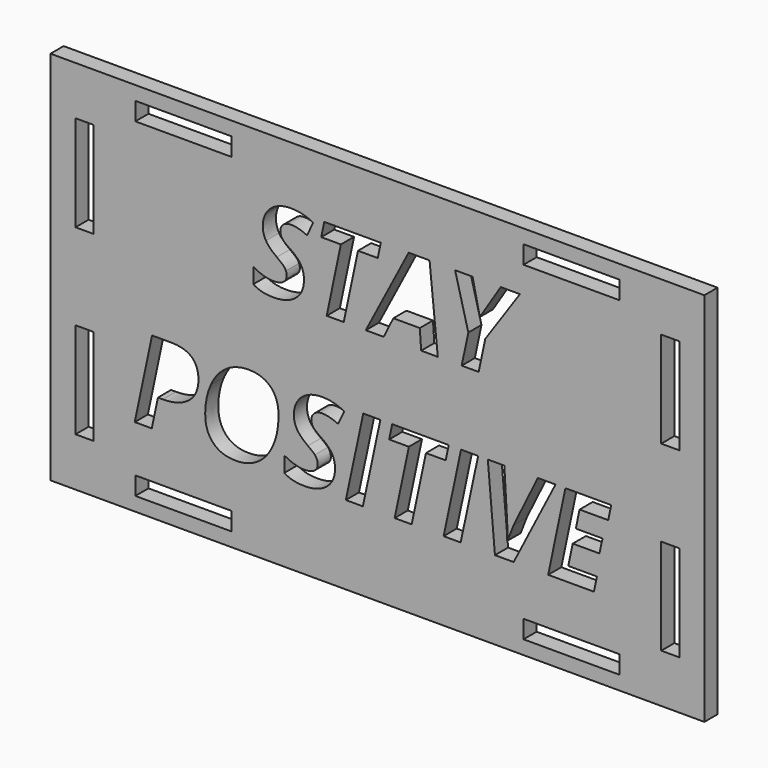
from build123d import *

# Parameters (mm, degrees)
F0_W     = 119.38
F0_H     = 68.58
F0_W_2   = 17.526
F0_H_2   = 3.302
F0_W_3   = 3.302
F0_H_3   = 17.526
F1_DEPTH = 3


with BuildPart() as f1:
    # F0 (on Front) → F1 (new body)
    with BuildSketch(Plane.XZ):
        Rectangle(F0_W, F0_H)
        with Locations((-35.433, -30.099)):
            Rectangle(F0_W_2, F0_H_2, mode=Mode.SUBTRACT)
        with Locations((-53.467, -16.637)):
            Rectangle(F0_W_3, F0_H_3, mode=Mode.SUBTRACT)
        with BuildLine():
            add(Edge.make_bspline(
                [(-33.9483112605, -6.0585155259), (-32.6803680163, -7.148128688), (-32.6803680163, -9.3240829005)],
                knots=[0, 0, 0, 1, 1, 1], degree=2))
            add(Edge.make_bspline(
                [(-32.6803680163, -9.3240829005), (-32.6803680163, -11.7912550452), (-34.4145871632, -13.1966269765)],
                knots=[0, 0, 0, 1, 1, 1], degree=2))
            add(Edge.make_bspline(
                [(-34.4145871632, -13.1966269765), (-36.14880631, -14.6019989077), (-39.1951422075, -14.6019989077)],
                knots=[0, 0, 0, 1, 1, 1], degree=2))
            Line((-39.1951422075, -14.6019989077), (-40.0753402273, -14.6019989077))
            Line((-40.0753402273, -14.6019989077), (-41.1878581706, -19.9191802541))
            Line((-41.1878581706, -19.9191802541), (-44.3061805232, -19.9191802541))
            Line((-44.3061805232, -19.9191802541), (-41.1485928314, -4.9689023639))
            Line((-41.1485928314, -4.9689023639), (-37.6899708725, -4.9689023639))
            add(Edge.make_bspline(
                [(-37.6899708725, -4.9689023639), (-35.2162545046, -4.9689023639), (-33.9483112605, -6.0585155259)],
                knots=[0, 0, 0, 1, 1, 1], degree=2))
        make_face(mode=Mode.SUBTRACT)
        with BuildLine():
            add(Edge.make_bspline(
                [(-19.4888501099, -6.2057605478), (-18.0573012859, -7.6782107668), (-18.0573012859, -10.328621161)],
                knots=[0, 0, 0, 1, 1, 1], degree=2))
            add(Edge.make_bspline(
                [(-18.0573012859, -10.328621161), (-18.0573012859, -13.2211678135), (-19.0700198254, -15.5067377645)],
                knots=[0, 0, 0, 1, 1, 1], degree=2))
            add(Edge.make_bspline(
                [(-19.0700198254, -15.5067377645), (-20.0827383649, -17.7923077156), (-21.8414983487, -18.9588155002)],
                knots=[0, 0, 0, 1, 1, 1], degree=2))
            add(Edge.make_bspline(
                [(-21.8414983487, -18.9588155002), (-23.6002583325, -20.1253232848), (-25.890736451, -20.1253232848)],
                knots=[0, 0, 0, 1, 1, 1], degree=2))
            add(Edge.make_bspline(
                [(-25.890736451, -20.1253232848), (-28.5084257292, -20.1253232848), (-29.9759677808, -18.6168798382)],
                knots=[0, 0, 0, 1, 1, 1], degree=2))
            add(Edge.make_bspline(
                [(-29.9759677808, -18.6168798382), (-31.4435098324, -17.1084363916), (-31.4435098324, -14.428576993)],
                knots=[0, 0, 0, 1, 1, 1], degree=2))
            add(Edge.make_bspline(
                [(-31.4435098324, -14.428576993), (-31.4435098324, -11.7192685901), (-30.4307912929, -9.4435149738)],
                knots=[0, 0, 0, 1, 1, 1], degree=2))
            add(Edge.make_bspline(
                [(-30.4307912929, -9.4435149738), (-29.4180727534, -7.1677613576), (-27.6380440442, -5.9505358432)],
                knots=[0, 0, 0, 1, 1, 1], degree=2))
            add(Edge.make_bspline(
                [(-27.6380440442, -5.9505358432), (-25.858015335, -4.7333103288), (-23.5282718774, -4.7333103288)],
                knots=[0, 0, 0, 1, 1, 1], degree=2))
            add(Edge.make_bspline(
                [(-23.5282718774, -4.7333103288), (-20.9203989339, -4.7333103288), (-19.4888501099, -6.2057605478)],
                knots=[0, 0, 0, 1, 1, 1], degree=2))
        make_face(mode=Mode.SUBTRACT)
        with BuildLine():
            add(Edge.make_bspline(
                [(-8.3538543427, -13.1966269765), (-7.7403334181, -14.1831686232), (-7.7403334181, -15.5018295971)],
                knots=[0, 0, 0, 1, 1, 1], degree=2))
            add(Edge.make_bspline(
                [(-7.7403334181, -15.5018295971), (-7.7403334181, -17.6385184705), (-9.2536850321, -18.8819208776)],
                knots=[0, 0, 0, 1, 1, 1], degree=2))
            add(Edge.make_bspline(
                [(-9.2536850321, -18.8819208776), (-10.767036646, -20.1253232848), (-13.3520048083, -20.1253232848)],
                knots=[0, 0, 0, 1, 1, 1], degree=2))
            add(Edge.make_bspline(
                [(-13.3520048083, -20.1253232848), (-15.6130339223, -20.1253232848), (-16.9938650166, -19.2025878142)],
                knots=[0, 0, 0, 1, 1, 1], degree=2))
            Line((-16.9938650166, -19.2025878142), (-16.9938650166, -16.4016602865))
            add(Edge.make_bspline(
                [(-16.9938650166, -16.4016602865), (-15.0207817231, -17.504361895), (-13.3323721387, -17.504361895)],
                knots=[0, 0, 0, 1, 1, 1], degree=2))
            add(Edge.make_bspline(
                [(-13.3323721387, -17.504361895), (-12.1871330795, -17.504361895), (-11.5425270947, -17.0708071083)],
                knots=[0, 0, 0, 1, 1, 1], degree=2))
            add(Edge.make_bspline(
                [(-11.5425270947, -17.0708071083), (-10.8979211099, -16.6372523215), (-10.8979211099, -15.8813945425)],
                knots=[0, 0, 0, 1, 1, 1], degree=2))
            add(Edge.make_bspline(
                [(-10.8979211099, -15.8813945425), (-10.8979211099, -15.4396594768), (-11.0369858528, -15.1075401496)],
                knots=[0, 0, 0, 1, 1, 1], degree=2))
            add(Edge.make_bspline(
                [(-11.0369858528, -15.1075401496), (-11.1760505957, -14.7754208224), (-11.4312753004, -14.4891110576)],
                knots=[0, 0, 0, 1, 1, 1], degree=2))
            add(Edge.make_bspline(
                [(-11.4312753004, -14.4891110576), (-11.686500005, -14.2028012928), (-12.6975824887, -13.4469435137)],
                knots=[0, 0, 0, 1, 1, 1], degree=2))
            add(Edge.make_bspline(
                [(-12.6975824887, -13.4469435137), (-14.111134699, -12.4325889184), (-14.6837542286, -11.4411391043)],
                knots=[0, 0, 0, 1, 1, 1], degree=2))
            add(Edge.make_bspline(
                [(-14.6837542286, -11.4411391043), (-15.2563737582, -10.4496892902), (-15.2563737582, -9.3044502309)],
                knots=[0, 0, 0, 1, 1, 1], degree=2))
            add(Edge.make_bspline(
                [(-15.2563737582, -9.3044502309), (-15.2563737582, -7.985789257), (-14.6215841082, -6.9485298805)],
                knots=[0, 0, 0, 1, 1, 1], degree=2))
            add(Edge.make_bspline(
                [(-14.6215841082, -6.9485298805), (-13.9867944582, -5.911270504), (-12.8153785062, -5.333742807)],
                knots=[0, 0, 0, 1, 1, 1], degree=2))
            add(Edge.make_bspline(
                [(-12.8153785062, -5.333742807), (-11.6439625542, -4.75621511), (-10.1224306613, -4.75621511)],
                knots=[0, 0, 0, 1, 1, 1], degree=2))
            add(Edge.make_bspline(
                [(-10.1224306613, -4.75621511), (-7.903938998, -4.75621511), (-6.0617401684, -5.7672975937)],
                knots=[0, 0, 0, 1, 1, 1], degree=2))
            Line((-6.0617401684, -5.7672975937), (-7.1775302233, -8.1493948369))
            add(Edge.make_bspline(
                [(-7.1775302233, -8.1493948369), (-8.7710485714, -7.3935370578), (-10.1224306613, -7.3935370578)],
                knots=[0, 0, 0, 1, 1, 1], degree=2))
            add(Edge.make_bspline(
                [(-10.1224306613, -7.3935370578), (-10.9699075651, -7.3935370578), (-11.5114420345, -7.8532687373)],
                knots=[0, 0, 0, 1, 1, 1], degree=2))
            add(Edge.make_bspline(
                [(-11.5114420345, -7.8532687373), (-12.052976504, -8.3130004168), (-12.052976504, -9.0688581959)],
                knots=[0, 0, 0, 1, 1, 1], degree=2))
            add(Edge.make_bspline(
                [(-12.052976504, -9.0688581959), (-12.052976504, -9.6938315111), (-11.7159490094, -10.1584713579)],
                knots=[0, 0, 0, 1, 1, 1], degree=2))
            add(Edge.make_bspline(
                [(-11.7159490094, -10.1584713579), (-11.3789215148, -10.6231112048), (-10.2042334512, -11.3920574303)],
                knots=[0, 0, 0, 1, 1, 1], degree=2))
            add(Edge.make_bspline(
                [(-10.2042334512, -11.3920574303), (-8.9673752672, -12.2100853298), (-8.3538543427, -13.1966269765)],
                knots=[0, 0, 0, 1, 1, 1], degree=2))
        make_face(mode=Mode.SUBTRACT)
        Polygon((-2.6554719951, -19.9191802541), (-5.7737943478, -19.9191802541), (-2.58348554, -4.9689023639), (0.5348368127, -4.9689023639), align=None, mode=Mode.SUBTRACT)
        with Locations((35.433, -30.099)):
            Rectangle(F0_W_2, F0_H_2, mode=Mode.SUBTRACT)
        Polygon((8.8558166058, -7.6062243117), (6.2577599972, -19.9191802541), (3.1394376445, -19.9191802541), (5.7374942532, -7.6062243117), (2.1381714956, -7.6062243117), (2.7009746904, -4.9689023639), (13.027758893, -4.9689023639), (12.4649556982, -7.6062243117), align=None, mode=Mode.SUBTRACT)
        Polygon((15.1971688823, -19.9191802541), (12.0788465297, -19.9191802541), (15.2691553375, -4.9689023639), (18.3874776902, -4.9689023639), align=None, mode=Mode.SUBTRACT)
        with BuildLine():
            Line((23.6719379206, -16.8630280218), (23.7439243757, -16.8630280218))
            add(Edge.make_bspline(
                [(23.7439243757, -16.8630280218), (24.5423196056, -14.6019989077), (24.8695307654, -13.9672092578)],
                knots=[0, 0, 0, 1, 1, 1], degree=2))
            Line((24.8695307654, -13.9672092578), (29.2868814224, -4.9689023639))
            Line((29.2868814224, -4.9689023639), (32.5164555694, -4.9689023639))
            Line((32.5164555694, -4.9689023639), (24.8695307654, -19.9191802541))
            Line((24.8695307654, -19.9191802541), (21.4534462573, -19.9191802541))
            Line((21.4534462573, -19.9191802541), (20.154417953, -4.9689023639))
            Line((20.154417953, -4.9689023639), (23.1713048461, -4.9689023639))
            Line((23.1713048461, -4.9689023639), (23.6915705902, -13.9672092578))
            add(Edge.make_bspline(
                [(23.6915705902, -13.9672092578), (23.7341080409, -14.428576993), (23.7341080409, -15.3284076824)],
                knots=[0, 0, 0, 1, 1, 1], degree=2))
            add(Edge.make_bspline(
                [(23.7341080409, -15.3284076824), (23.7144753713, -16.3820276169), (23.6719379206, -16.8630280218)],
                knots=[0, 0, 0, 1, 1, 1], degree=2))
        make_face(mode=Mode.SUBTRACT)
        Polygon((40.0750333602, -17.3014909759), (39.5220465002, -19.9191802541), (31.1683455911, -19.9191802541), (34.3259332829, -4.9689023639), (42.6927226385, -4.9689023639), (42.1397357784, -7.5669589725), (36.904357222, -7.5669589725), (36.2172137865, -10.8488869051), (41.0959321787, -10.8488869051), (40.5331289839, -13.4469435137), (35.6576827032, -13.4469435137), (34.8396548038, -17.3014909759), align=None, mode=Mode.SUBTRACT)
        with Locations((53.467, -16.637)):
            Rectangle(F0_W_3, F0_H_3, mode=Mode.SUBTRACT)
        with Locations((-53.467, 16.637)):
            Rectangle(F0_W_3, F0_H_3, mode=Mode.SUBTRACT)
        with BuildLine():
            add(Edge.make_bspline(
                [(-14.0244237416, 15.2838323706), (-13.410902817, 14.2972907238), (-13.410902817, 12.9786297499)],
                knots=[0, 0, 0, 1, 1, 1], degree=2))
            add(Edge.make_bspline(
                [(-13.410902817, 12.9786297499), (-13.410902817, 10.8419408766), (-14.924254431, 9.5985384694)],
                knots=[0, 0, 0, 1, 1, 1], degree=2))
            add(Edge.make_bspline(
                [(-14.924254431, 9.5985384694), (-16.437606045, 8.3551360623), (-19.0225742072, 8.3551360623)],
                knots=[0, 0, 0, 1, 1, 1], degree=2))
            add(Edge.make_bspline(
                [(-19.0225742072, 8.3551360623), (-21.2836033213, 8.3551360623), (-22.6644344155, 9.2778715328)],
                knots=[0, 0, 0, 1, 1, 1], degree=2))
            Line((-22.6644344155, 9.2778715328), (-22.6644344155, 12.0787990605))
            add(Edge.make_bspline(
                [(-22.6644344155, 12.0787990605), (-20.6913511221, 10.9760974521), (-19.0029415376, 10.9760974521)],
                knots=[0, 0, 0, 1, 1, 1], degree=2))
            add(Edge.make_bspline(
                [(-19.0029415376, 10.9760974521), (-17.8577024784, 10.9760974521), (-17.2130964936, 11.4096522388)],
                knots=[0, 0, 0, 1, 1, 1], degree=2))
            add(Edge.make_bspline(
                [(-17.2130964936, 11.4096522388), (-16.5684905089, 11.8432070255), (-16.5684905089, 12.5990648046)],
                knots=[0, 0, 0, 1, 1, 1], degree=2))
            add(Edge.make_bspline(
                [(-16.5684905089, 12.5990648046), (-16.5684905089, 13.0407998703), (-16.7075552518, 13.3729191975)],
                knots=[0, 0, 0, 1, 1, 1], degree=2))
            add(Edge.make_bspline(
                [(-16.7075552518, 13.3729191975), (-16.8466199947, 13.7050385246), (-17.1018446993, 13.9913482894)],
                knots=[0, 0, 0, 1, 1, 1], degree=2))
            add(Edge.make_bspline(
                [(-17.1018446993, 13.9913482894), (-17.3570694039, 14.2776580542), (-18.3681518877, 15.0335158333)],
                knots=[0, 0, 0, 1, 1, 1], degree=2))
            add(Edge.make_bspline(
                [(-18.3681518877, 15.0335158333), (-19.7817040979, 16.0478704286), (-20.3543236275, 17.0393202428)],
                knots=[0, 0, 0, 1, 1, 1], degree=2))
            add(Edge.make_bspline(
                [(-20.3543236275, 17.0393202428), (-20.9269431571, 18.0307700569), (-20.9269431571, 19.1760091161)],
                knots=[0, 0, 0, 1, 1, 1], degree=2))
            add(Edge.make_bspline(
                [(-20.9269431571, 19.1760091161), (-20.9269431571, 20.49467009), (-20.2921535072, 21.5319294665)],
                knots=[0, 0, 0, 1, 1, 1], degree=2))
            add(Edge.make_bspline(
                [(-20.2921535072, 21.5319294665), (-19.6573638572, 22.569188843), (-18.4859479052, 23.14671654)],
                knots=[0, 0, 0, 1, 1, 1], degree=2))
            add(Edge.make_bspline(
                [(-18.4859479052, 23.14671654), (-17.3145319532, 23.724244237), (-15.7930000602, 23.724244237)],
                knots=[0, 0, 0, 1, 1, 1], degree=2))
            add(Edge.make_bspline(
                [(-15.7930000602, 23.724244237), (-13.5745083969, 23.724244237), (-11.7323095674, 22.7131617533)],
                knots=[0, 0, 0, 1, 1, 1], degree=2))
            Line((-11.7323095674, 22.7131617533), (-12.8480996222, 20.3310645101))
            add(Edge.make_bspline(
                [(-12.8480996222, 20.3310645101), (-14.4416179703, 21.0869222892), (-15.7930000602, 21.0869222892)],
                knots=[0, 0, 0, 1, 1, 1], degree=2))
            add(Edge.make_bspline(
                [(-15.7930000602, 21.0869222892), (-16.640476964, 21.0869222892), (-17.1820114335, 20.6271906097)],
                knots=[0, 0, 0, 1, 1, 1], degree=2))
            add(Edge.make_bspline(
                [(-17.1820114335, 20.6271906097), (-17.7235459029, 20.1674589302), (-17.7235459029, 19.4116011512)],
                knots=[0, 0, 0, 1, 1, 1], degree=2))
            add(Edge.make_bspline(
                [(-17.7235459029, 19.4116011512), (-17.7235459029, 18.786627836), (-17.3865184083, 18.3219879891)],
                knots=[0, 0, 0, 1, 1, 1], degree=2))
            add(Edge.make_bspline(
                [(-17.3865184083, 18.3219879891), (-17.0494909138, 17.8573481422), (-15.8748028502, 17.0884019167)],
                knots=[0, 0, 0, 1, 1, 1], degree=2))
            add(Edge.make_bspline(
                [(-15.8748028502, 17.0884019167), (-14.6379446662, 16.2703740173), (-14.0244237416, 15.2838323706)],
                knots=[0, 0, 0, 1, 1, 1], degree=2))
        make_face(mode=Mode.SUBTRACT)
        Polygon((-3.5520305729, 20.8742350354), (-6.1500871816, 8.5612790929), (-9.2684095342, 8.5612790929), (-6.6703529256, 20.8742350354), (-10.2696756832, 20.8742350354), (-9.7068724883, 23.5115569832), (0.6199117142, 23.5115569832), (0.0571085194, 20.8742350354), align=None, mode=Mode.SUBTRACT)
        with Locations((-35.433, 30.099)):
            Rectangle(F0_W_2, F0_H_2, mode=Mode.SUBTRACT)
        Polygon((7.9821628092, 8.5612790929), (7.7367544394, 12.1213365113), (2.9005734979, 12.1213365113), (1.1434495699, 8.5612790929), (-2.1286620279, 8.5612790929), (5.7015010256, 23.5737271035), (9.5167831486, 23.5737271035), (11.018682372, 8.5612790929), align=None, mode=Mode.SUBTRACT)
        Polygon((17.3698509833, 23.5115569832), (18.6885119572, 17.4581505273), (22.513610415, 23.5115569832), (26.011497713, 23.5115569832), (19.6930502177, 14.2776580542), (18.4758247033, 8.5612790929), (15.3771350202, 8.5612790929), (16.5943605346, 14.2776580542), (14.1795421754, 23.5115569832), align=None, mode=Mode.SUBTRACT)
        with Locations((53.467, 16.637)):
            Rectangle(F0_W_3, F0_H_3, mode=Mode.SUBTRACT)
        with Locations((35.433, 30.099)):
            Rectangle(F0_W_2, F0_H_2, mode=Mode.SUBTRACT)
    extrude(amount=F1_DEPTH)


solid = f1.part
